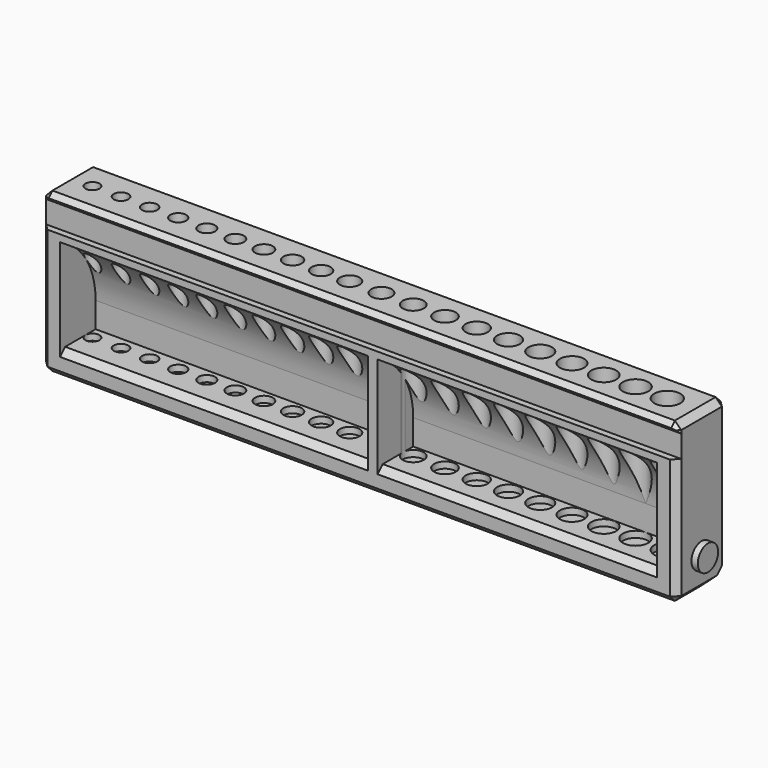
from build123d import *

# Parameters (mm, degrees)
F0_W          = 100
F0_H          = 10
F2_DEPTH      = 25
F3_START      = 3
F1_R          = 2.05
F1_R_2        = 2
F1_R_3        = 1.95
F1_R_4        = 1.9
F1_R_5        = 1.85
F1_R_6        = 1.8
F1_R_7        = 1.75
F1_R_8        = 1.7
F1_R_9        = 1.65
F1_R_10       = 1.6
F1_R_11       = 1.55
F1_R_12       = 1.5
F1_R_13       = 1.45
F1_R_14       = 1.4
F1_R_15       = 1.35
F1_R_16       = 1.3
F1_R_17       = 1.25
F1_R_18       = 1.2
F1_R_19       = 1.15
F1_R_20       = 1.1
F3_DEPTH      = 37
F5_START      = -3
F5_DEPTH      = 44
F6_START      = -48.5
F6_DEPTH      = 48.5
F7_SIZE       = 1
F8_R          = 2
F9_DEPTH      = 2
F9_DEPTH_BACK = 1
F10_START     = -99
F10_DEPTH     = 2
F11_T1_DEPTH  = 123
F13_START     = 9
F13_DEPTH     = 16
F14_T4_DEPTH  = 103.143366


# Not quite as in the source:
# - a fillet or chamfer that OpenCascade refuses, or shapes differently, is made with other operations: its cross-section is extruded or revolved along the edge and cut away or added


with BuildPart() as f2:
    # F0 (on Top) → F2 (new body)
    with BuildSketch(Plane.XY):
        with Locations((-50, -5)):
            Rectangle(F0_W, F0_H)
    extrude(amount=F2_DEPTH)

    # F1 (on Top) → F3 (cut)
    with BuildSketch(Plane.XY.offset(F3_START)):
        with Locations((-5.4, -5)):
            Circle(F1_R)
        with Locations((-10.4, -5)):
            Circle(F1_R_2)
        with Locations((-15.4, -5)):
            Circle(F1_R_3)
        with Locations((-20.4, -5)):
            Circle(F1_R_4)
        with Locations((-25.4, -5)):
            Circle(F1_R_5)
        with Locations((-30.4, -5)):
            Circle(F1_R_6)
        with Locations((-35.4, -5)):
            Circle(F1_R_7)
        with Locations((-40.4, -5)):
            Circle(F1_R_8)
        with Locations((-45.4, -5)):
            Circle(F1_R_9)
        with Locations((-50.4, -5)):
            Circle(F1_R_10)
        with Locations((-55.4, -5)):
            Circle(F1_R_11)
        with Locations((-59.9, -5)):
            Circle(F1_R_12)
        with Locations((-64.4, -5)):
            Circle(F1_R_13)
        with Locations((-68.9, -5)):
            Circle(F1_R_14)
        with Locations((-73.4, -5)):
            Circle(F1_R_15)
        with Locations((-77.9, -5)):
            Circle(F1_R_16)
        with Locations((-82.4, -5)):
            Circle(F1_R_17)
        with Locations((-86.9, -5)):
            Circle(F1_R_18)
        with Locations((-91.4, -5)):
            Circle(F1_R_19)
        with Locations((-95.9, -5)):
            Circle(F1_R_20)
    extrude(amount=F3_DEPTH, mode=Mode.SUBTRACT)

    # F4 (on Right) → F5 (cut)
    with BuildSketch(Plane.YZ.offset(F5_START)):
        with BuildLine():
            Line((-13, 19.83216), (-13, 4))
            Line((-13, 4), (-3, 4))
            Line((-3, 4), (-3, 8))
            ThreePointArc((-3, 8), (-5.834849, 15.745967), (-13, 19.83216))
        make_face()
        with BuildLine():
            ThreePointArc((-15, 20), (-13.996485, 19.957966), (-13, 19.83216))
            Line((-13, 19.83216), (-13, 20))
            Line((-13, 20), (-15, 20))
        make_face()
    extrude(amount=-F5_DEPTH, mode=Mode.SUBTRACT)

    # F4 (on Right) → F6 (cut)
    with BuildSketch(Plane.YZ.offset(F6_START)):
        with BuildLine():
            Line((-13, 19.83216), (-13, 4))
            Line((-13, 4), (-3, 4))
            Line((-3, 4), (-3, 8))
            ThreePointArc((-3, 8), (-5.834849, 15.745967), (-13, 19.83216))
        make_face()
        with BuildLine():
            ThreePointArc((-15, 20), (-13.996485, 19.957966), (-13, 19.83216))
            Line((-13, 19.83216), (-13, 20))
            Line((-13, 20), (-15, 20))
        make_face()
    extrude(amount=-F6_DEPTH, mode=Mode.SUBTRACT)

    # F7
    f7_edges = [f2.edges().sort_by_distance(p)[0] for p in [
        (-50, -10, 25),
        (-100, -5, 25),
        (-50, 0, 25),
        (0, -5, 25),
        (0, -10, 12.5),
        (0, 0, 12.5),
        (0, -5, 0),
        (-50, -10, 0),
        (-100, -10, 12.5),
        (-72.75, -10, 4),
        (-25, -10, 4),
        (-100, -5, 0),
        (-100, 0, 12.5),
    ]]
    chamfer(f7_edges, length=F7_SIZE)

    # F8 (on Right) → F9 (join, two sides)
    with BuildSketch(Plane.YZ) as f9_sk:
        with Locations((-5, 5)):
            Circle(F8_R)
    extrude(amount=-F9_DEPTH)
    extrude(f9_sk.sketch, amount=F9_DEPTH_BACK)

    # F8 (on Right) → F10 (join)
    with BuildSketch(Plane.YZ.offset(F10_START)):
        with Locations((-5, 5)):
            Circle(F8_R)
    extrude(amount=-F10_DEPTH)

    # F11: fillet of radius 5 on 1 edges, made by hand

    # F11_s2 → F11_t1 (cut)
    with BuildSketch(Plane.YZ.offset(-111.5)):
        with BuildLine():
            ThreePointArc((0, 5), (-1.464466, 1.464466), (-5, 0))
            Line((-5, 0), (0, 0))
            Line((0, 0), (0, 5))
        make_face()
    extrude(amount=F11_T1_DEPTH, mode=Mode.SUBTRACT)

    # F12 (on Front) → F13 (cut)
    with BuildSketch(Plane.XZ.offset(F13_START)):
        Polygon((-105, 20), (0, 20), (5, 20), (5, 23.5), (-105, 23.5), align=None)
    extrude(amount=F13_DEPTH, mode=Mode.SUBTRACT)

    # F14: chamfer of 1 on 1 edges, made by hand


with BuildPart() as f14_tool2:
    # F14_s3 → F14_t4 (new body)
    with BuildSketch(Plane.YZ.offset(1.571683)):
        Polygon((-9, 23.5), (-10, 24.5), (-10, 23.5), align=None)
    extrude(amount=-F14_T4_DEPTH)

    split(bisect_by=Plane.XZ.offset(9), keep=Keep.TOP)


with BuildPart() as f2_1:
    add(f2.part)

    # F14_t1: cut F14_tool2
    add(f14_tool2.part, mode=Mode.SUBTRACT)


solid = f2_1.part
